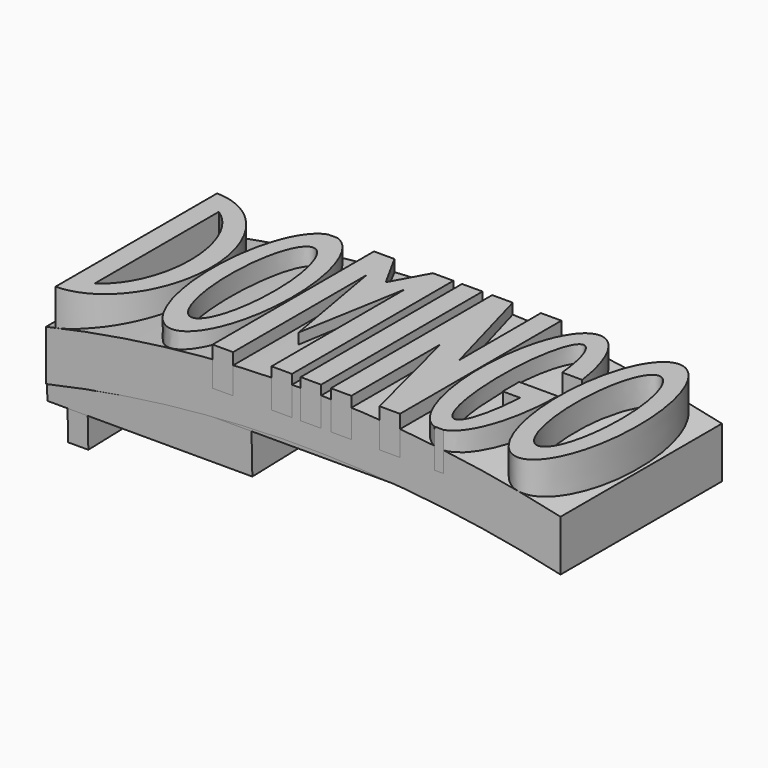
from build123d import *

# Parameters (mm, degrees)
F1_DEPTH  = 20
F3_DEPTH  = 5.08
F5_DEPTH  = 50.8
F7_DEPTH  = 3.81
F10_W     = 2
F10_H     = 2.5
F11_DEPTH = 5
F12_W     = 2
F12_H     = 17.5
F12_H_2   = 2.5
F13_DEPTH = 2
F16_DEPTH = 3.81
F18_DEPTH = 3.81
F19_W     = 2.032
F19_H     = 20
F20_DEPTH = 3.81
F22_DEPTH = 3.81
F24_DEPTH = 3.81
F26_DEPTH = 3.81
F27_W     = 20.32
F27_H     = 20
F28_DEPTH = 4


# Not quite as in the source:
# - a feature names something its author has since deleted; it is built from what else it names


with BuildPart() as f1:
    # F0 (on Front) → F1 (new body)
    with BuildSketch(Plane.XZ):
        with BuildLine():
            ThreePointArc((-30.0034920961, 27.8728295863), (-4.5009065508, 30.7307358305), (20.9965079039, 27.8270564899))
            Line((20.9965079039, 27.8270564899), (20.9965079039, 32.8728295863))
            ThreePointArc((20.9965079039, 32.8728295863), (-4.5034920961, 35.7536211884), (-30.0034920961, 32.8728295863))
            Line((-30.0034920961, 32.8728295863), (-30.0034920961, 27.8728295863))
        make_face()
    extrude(amount=F1_DEPTH)


with BuildPart() as f3:
    # F2 (on Top) → F3 (new body)
    with BuildSketch(Plane.XY):
        with BuildLine():
            ThreePointArc((-23.3267513332, 4.2796317959), (-19.3655130555, 8.0896317959), (-23.3267513332, 11.8996317959))
            Line((-23.3267513332, 11.8996317959), (-23.3267513332, 4.2796317959))
        make_face()
    extrude(amount=F3_DEPTH)


with BuildPart() as f5:
    # F4 (on face) → F5 (new body)
    with BuildSketch(Plane(origin=(-30.0034920961, 0, 0), x_dir=(0, -1, 0), z_dir=(-1, 0, 0))):
        Polygon((19.9419356, 30.3334933491), (20, 32.8728295863), (0, 32.8728295863), (-0.0516119673, 30.8414851534), align=None)
    extrude(amount=-F5_DEPTH)


with BuildPart() as f7:
    # F6 (on face) → F7 (new body)
    with BuildSketch(Plane.XY.offset(32.8728295863)):
        with BuildLine():
            add(Edge.make_bspline(
                [(-21.6551118063, -10), (-21.6551118063, 0), (-29.0568315381, 0)],
                knots=[1.5707963268, 1.5707963268, 1.5707963268, 3.1415926536, 3.1415926536, 3.1415926536], degree=2, weights=[1, 0.7071067812, 1]))
            Line((-29.0568315381, 0), (-29.0568315381, -1.7085451704))
            add(Edge.make_bspline(
                [(-27.0248315381, -2.3251747334), (-28.0015928656, -1.7085451704), (-29.0568315381, -1.7085451704)],
                knots=[5.895087864, 5.895087864, 5.895087864, 6.2831853072, 6.2831853072, 6.2831853072], degree=2, weights=[1, 0.9812315516, 1]))
            add(Edge.make_bspline(
                [(-23.687250518, -10), (-23.687250518, -4.4321900993), (-27.0248315381, -2.3251747334)],
                knots=[4.7123889804, 4.7123889804, 4.7123889804, 5.895087864, 5.895087864, 5.895087864], degree=2, weights=[1, 0.8301891459, 1]))
            Line((-23.687250518, -10), (-21.6551118063, -10))
        make_face()
        with BuildLine():
            add(Edge.make_bspline(
                [(-27.0248315381, -2.3251747334), (-28.0015928656, -1.7085451704), (-29.0568315381, -1.7085451704)],
                knots=[5.895087864, 5.895087864, 5.895087864, 6.2831853072, 6.2831853072, 6.2831853072], degree=2, weights=[1, 0.9812315516, 1]))
            Line((-29.0568315381, -1.7085451704), (-29.0568315381, -18.2914548296))
            add(Edge.make_bspline(
                [(-29.0568315381, -18.2914548296), (-28.0015928656, -18.2914548296), (-27.0248315381, -17.6748252666)],
                knots=[3.1415926536, 3.1415926536, 3.1415926536, 3.5296900968, 3.5296900968, 3.5296900968], degree=2, weights=[1, 0.9812315516, 1]))
            Line((-27.0248315381, -17.6748252666), (-27.0248315381, -2.3251747334))
        make_face()
        with BuildLine():
            add(Edge.make_bspline(
                [(-29.0568315381, -20), (-21.6551118063, -20), (-21.6551118063, -10)],
                knots=[0, 0, 0, 1.5707963268, 1.5707963268, 1.5707963268], degree=2, weights=[1, 0.7071067812, 1]))
            Line((-21.6551118063, -10), (-23.687250518, -10))
            add(Edge.make_bspline(
                [(-27.0248315381, -17.6748252666), (-23.687250518, -15.5678099007), (-23.687250518, -10)],
                knots=[3.5296900968, 3.5296900968, 3.5296900968, 4.7123889804, 4.7123889804, 4.7123889804], degree=2, weights=[1, 0.8301891459, 1]))
            add(Edge.make_bspline(
                [(-29.0568315381, -18.2914548296), (-28.0015928656, -18.2914548296), (-27.0248315381, -17.6748252666)],
                knots=[3.1415926536, 3.1415926536, 3.1415926536, 3.5296900968, 3.5296900968, 3.5296900968], degree=2, weights=[1, 0.9812315516, 1]))
            Line((-29.0568315381, -18.2914548296), (-29.0568315381, -20))
        make_face()
    extrude(amount=F7_DEPTH)


with BuildPart() as f8_1:
    # F8: copy of F7
    add(f7.part.moved(Location((9.3726, -0.1524, 0))))


with BuildPart() as f11:
    # F10 (on face) → F11 (new body)
    with BuildSketch(Plane(origin=(0, -0.7830750584, 30.820277603), x_dir=(1, 0, 0), z_dir=(0, 0.0253995902, -0.9996773784))):
        with Locations((-27.0034920961, 17.9150435992)):
            Rectangle(F10_W, F10_H)
    extrude(amount=F11_DEPTH)



with BuildPart() as f11b:
    # F10 (on face) → F11, piece 2 (new body)
    with BuildSketch(Plane(origin=(0, -0.7830750584, 30.820277603), x_dir=(1, 0, 0), z_dir=(0, 0.0253995902, -0.9996773784))):
        with Locations((-27.0034920961, 0.4150435992)):
            Rectangle(F10_W, F10_H)
    extrude(amount=F11_DEPTH)


with BuildPart() as f11_1:
    add(f11.part)

    add(f11b.part)  # F13 merges F11b
    # F12 (on face) → F13 (join)
    with BuildSketch(Plane(origin=(0, -0.6560771074, 25.8218907112), x_dir=(1, 0, 0), z_dir=(0, 0.0253995902, -0.9996773784))):
        with Locations((-27.0034920961, 7.9150435992)):
            Rectangle(F12_W, F12_H)
        with Locations((-27.0034920961, 17.9150435992)):
            Rectangle(F12_W, F12_H_2)
    extrude(amount=F13_DEPTH)


with BuildPart() as f16:
    # F15 (on face) → F16 (new body)
    with BuildSketch(Plane.XY.offset(32.8728295863)):
        with BuildLine():
            Line((-17.1534108904, 0), (-18.0166152331, 0))
            add(Edge.make_bspline(
                [(-18.0166152331, 0), (-24.2708850663, -1.7441122403), (-20.927949064, -15.252977549), (-17.5850130618, -28.7618428577), (-14.2420770595, -15.252977549), (-10.8991410572, -1.7441122403), (-17.1534108904, 0)],
                knots=[0.109598277, 0.109598277, 0.109598277, 2.1309278614, 2.1309278614, 4.1522574458, 4.1522574458, 6.1735870302, 6.1735870302, 6.1735870302], degree=2, weights=[1, 0.5312976367, 1, 0.5312976367, 1, 0.5312976367, 1]))
        make_face()
        with BuildLine():
            add(Edge.make_bspline(
                [(-17.5850130618, -2.4325794168), (-21.4297780105, -2.4325794168), (-19.5073955361, -13.693712065), (-17.5850130618, -24.9548447132), (-15.6626305874, -13.693712065), (-13.740248113, -2.4325794168), (-17.5850130618, -2.4325794168)],
                knots=[0, 0, 0, 2.0943951024, 2.0943951024, 4.1887902048, 4.1887902048, 6.2831853072, 6.2831853072, 6.2831853072], degree=2, weights=[1, 0.5, 1, 0.5, 1, 0.5, 1]))
        make_face(mode=Mode.SUBTRACT)
    extrude(amount=F16_DEPTH)


with BuildPart() as f18:
    # F17 (on face) → F18 (new body)
    with BuildSketch(Plane.XY.offset(32.8728295863)):
        Polygon((-11.4650256, 0), (-13.4970256, 0), (-13.4970256, -20), (-11.4650256, -20), (-11.4650256, -3.4674343187), (-9.5600256, -14.2712261851), (-7.6550256, -3.4674343187), (-7.6550256, -20), (-5.6230256, -20), (-5.6230256, 0), (-7.6550256, 0), (-9.5600256, -3.4674343187), align=None)
    extrude(amount=F18_DEPTH)


with BuildPart() as f20:
    # F19 (on face) → F20 (new body)
    with BuildSketch(Plane.XY.offset(32.8728295863)):
        with Locations((-3.7531224609, -10)):
            Rectangle(F19_W, F19_H)
    extrude(amount=F20_DEPTH)


with BuildPart() as f22:
    # F21 (on face) → F22 (new body)
    with BuildSketch(Plane.XY.offset(32.8728295863)):
        Polygon((0.2567827138, 0), (-1.7752172862, 0), (-1.7752172862, -20), (0.2567827138, -20), (0.2567827138, -8.9636895339), (3.0499742861, -20), (5.0819742861, -20), (5.0819742861, 0), (3.0499742861, 0), (3.0499742861, -10.1300096139), align=None)
    extrude(amount=F22_DEPTH)


with BuildPart() as f24:
    # F23 (on face) → F24 (new body)
    with BuildSketch(Plane.XY.offset(32.8728295863)):
        with BuildLine():
            Line((10.5636952101, -6.7442721921), (12.5413244548, -6.7442721921))
            add(Edge.make_bspline(
                [(12.5413244548, -6.7442721921), (11.6456273989, -0.0633203983), (8.9469710365, -0.0633203983)],
                knots=[5.0507111283, 5.0507111283, 5.0507111283, 6.2831853072, 6.2831853072, 6.2831853072], degree=2, weights=[1, 0.8160590728, 1]))
            Line((8.9469710365, -0.0633203983), (8.9469710365, -2.0953203983))
            add(Edge.make_bspline(
                [(10.5636952101, -6.7442721921), (10.0882843347, -2.0953203983), (8.9469710365, -2.0953203983)],
                knots=[5.1420330138, 5.1420330138, 5.1420330138, 6.2831853072, 6.2831853072, 6.2831853072], degree=2, weights=[1, 0.8415899282, 1]))
        make_face()
        with BuildLine():
            add(Edge.make_bspline(
                [(9.3750887987, -20), (12.7573222927, -18.9963194219), (12.7573222927, -10.0633203983)],
                knots=[3.2541869127, 3.2541869127, 3.2541869127, 4.7123889804, 4.7123889804, 4.7123889804], degree=2, weights=[1, 0.7457735944, 1]))
            Line((12.7573222927, -10.0633203983), (10.7253222927, -10.0633203983))
            add(Edge.make_bspline(
                [(10.6665224551, -12.0953203983), (10.7253222927, -11.0963993855), (10.7253222927, -10.0633203983)],
                knots=[4.4545205103, 4.4545205103, 4.4545205103, 4.7123889804, 4.7123889804, 4.7123889804], degree=2, weights=[1, 0.9916994901, 1]))
            add(Edge.make_bspline(
                [(8.9469710365, -18.0313203983), (10.3171096068, -18.0313203983), (10.6665224551, -12.0953203983)],
                knots=[3.1415926536, 3.1415926536, 3.1415926536, 4.4545205103, 4.4545205103, 4.4545205103], degree=2, weights=[1, 0.7921553132, 1]))
            Line((8.9469710365, -18.0313203983), (8.9469710365, -20))
            Line((8.9469710365, -20), (9.3750887987, -20))
        make_face()
        with BuildLine():
            add(Edge.make_bspline(
                [(10.6665224551, -12.0953203983), (10.7253222927, -11.0963993855), (10.7253222927, -10.0633203983)],
                knots=[4.4545205103, 4.4545205103, 4.4545205103, 4.7123889804, 4.7123889804, 4.7123889804], degree=2, weights=[1, 0.9916994901, 1]))
            Line((10.7253222927, -10.0633203983), (8.9469710365, -10.0633203983))
            Line((8.9469710365, -10.0633203983), (8.9469710365, -12.0953203983))
            Line((8.9469710365, -12.0953203983), (10.6665224551, -12.0953203983))
        make_face()
        with BuildLine():
            Line((8.9469710365, -2.0953203983), (8.9469710365, -0.0633203983))
            add(Edge.make_bspline(
                [(8.9469710365, -0.0633203983), (5.345312344, -0.0633203983), (5.1426563861, -9.5006464327), (4.9400004281, -18.937972467), (8.5188532743, -20)],
                knots=[0, 0, 0, 1.5144991972, 1.5144991972, 3.0289983945, 3.0289983945, 3.0289983945], degree=2, weights=[1, 0.7267280773, 1, 0.7267280773, 1]))
            Line((8.5188532743, -20), (8.9469710365, -20))
            Line((8.9469710365, -20), (8.9469710365, -18.0313203983))
            add(Edge.make_bspline(
                [(8.9469710365, -2.0953203983), (7.1686197803, -2.0953203983), (7.1686197803, -10.0633203983), (7.1686197803, -18.0313203983), (8.9469710365, -18.0313203983)],
                knots=[0, 0, 0, 1.5707963268, 1.5707963268, 3.1415926536, 3.1415926536, 3.1415926536], degree=2, weights=[1, 0.7071067812, 1, 0.7071067812, 1]))
        make_face()
    extrude(amount=F24_DEPTH)


with BuildPart() as f26:
    # F25 (on face) → F26 (new body)
    with BuildSketch(Plane.XY.offset(32.8728295863)):
        with BuildLine():
            add(Edge.make_bspline(
                [(16.7731456459, -20), (20.7228456459, -20), (20.7228456459, -10), (20.7228456459, 0), (16.7731456459, 0)],
                knots=[3.1415926536, 3.1415926536, 3.1415926536, 4.7123889804, 4.7123889804, 6.2831853072, 6.2831853072, 6.2831853072], degree=2, weights=[1, 0.7071067812, 1, 0.7071067812, 1]))
            add(Edge.make_bspline(
                [(16.7731456459, 0), (12.8234456459, 0), (12.8234456459, -10), (12.8234456459, -20), (16.7731456459, -20)],
                knots=[0, 0, 0, 1.5707963268, 1.5707963268, 3.1415926536, 3.1415926536, 3.1415926536], degree=2, weights=[1, 0.7071067812, 1, 0.7071067812, 1]))
        make_face()
        with BuildLine():
            add(Edge.make_bspline(
                [(16.7731456459, -2.4943), (12.923662726, -2.4943), (14.8484041859, -13.75285), (16.7731456459, -25.0114), (18.6978871058, -13.75285), (20.6226285657, -2.4943), (16.7731456459, -2.4943)],
                knots=[0, 0, 0, 2.0943951024, 2.0943951024, 4.1887902048, 4.1887902048, 6.2831853072, 6.2831853072, 6.2831853072], degree=2, weights=[1, 0.5, 1, 0.5, 1, 0.5, 1]))
        make_face(mode=Mode.SUBTRACT)
    extrude(amount=F26_DEPTH)


with BuildPart() as f28:
    # F27 (on face) → F28 (new body)
    with BuildSketch(Plane(origin=(0, -0.7830750584, 30.820277603), x_dir=(1, 0, 0), z_dir=(0, 0.0253995902, -0.9996773784))):
        with Locations((-19.8434920961, 9.1650435992)):
            Rectangle(F27_W, F27_H)
    extrude(amount=F28_DEPTH)


solid = Compound([f1.part, f5.part, f7.part, f11_1.part, f16.part, f18.part, f20.part, f22.part, f24.part, f26.part, f28.part])
